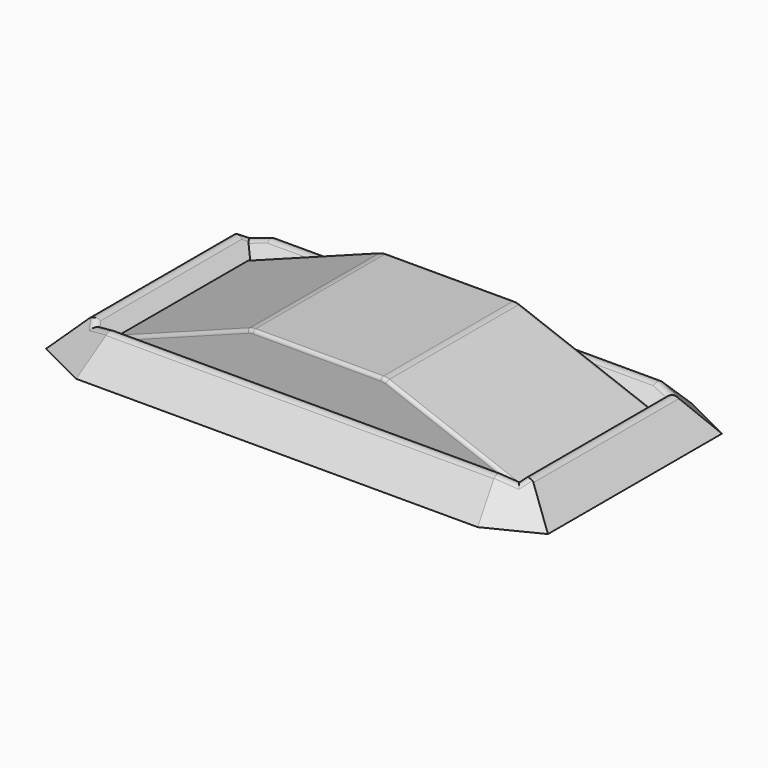
from build123d import *

# Parameters (mm, degrees)
F0_W         = 30.48
F0_H         = 12.7
F1_DEPTH     = 2.54
F2_T1_DEPTH  = 34.8362243683
F3_SIZE      = 2.53999
F4_SIZE      = 2.53999
F5_T4_DEPTH  = 37.0120747894
F5_T10_DEPTH = 19.2320747894
F5_T16_DEPTH = 37.0120747894
F5_T22_DEPTH = 19.2320747894
F6_DEPTH     = 5.08
F7_SIZE2     = 3.80999
F7_SIZE      = 10.15999
F8_T1_DEPTH  = 12.31902
F8_T6_DEPTH  = 12.565371882
F8_T12_DEPTH = 12.565371882
F8_T18_DEPTH = 12.565371882
F8_T24_DEPTH = 12.565371882
F9_T1_DEPTH  = 12.7000000001
F9_T4_ANGLE  = 20.556014319
F9_T6_ANGLE  = 20.556014319
F9_T8_ANGLE  = 20.556014319
F9_T10_ANGLE = 20.556014319
F10_R        = 0.508


# Not quite as in the source:
# - a fillet or chamfer that OpenCascade refuses, or shapes differently, is made with other operations: its cross-section is extruded or revolved along the edge and cut away or added
# - a fillet or chamfer is up to 0.001 mm smaller than in the source, because OpenCascade refuses the exact size


with BuildPart() as f1:
    # F0 (on Top) → F1 (new body)
    with BuildSketch(Plane.XY):
        Polygon((-11.5051504266, -16.4258122915), (-41.9851504266, -16.4258122915), (-47.0651499927, -18.9658166862), (-47.0651499927, -34.2058166862), (-41.9851488709, -36.7458122915), (-11.5051488709, -36.7458122915), (-6.4251502044, -34.2058166862), (-6.4251502044, -18.9658166862), align=None)
        with Locations((-26.7451504266, -26.5858122915)):
            Rectangle(F0_W, F0_H, mode=Mode.SUBTRACT)
    extrude(amount=F1_DEPTH)

    # F2: chamfer of 3.81 on 2 edges, made by hand

    # F2_s2 → F2_t1 (cut)
    with BuildSketch(Plane.XZ.offset(9.167704502)):
        Polygon((-47.0651499927, -1.27), (-43.2551499927, 2.54), (-47.0651499927, 2.54), align=None)
        Polygon((-6.4251502044, -1.27), (-10.2351502044, 2.54), (-6.4251502044, 2.54), align=None)
    extrude(amount=F2_T1_DEPTH, mode=Mode.SUBTRACT)

    # F3 (size 2.54 in the source; OpenCascade refuses exactly that, so slightly less here)
    f3_edges = [f1.edges().sort_by_distance(p)[0] for p in [
        (-42.620149, -36.428313, 2.54),
        (-42.62015, -16.743313, 2.54),
        (-10.87015, -16.743313, 2.54),
        (-10.87015, -36.428313, 2.54),
    ]]
    chamfer(f3_edges, length=F3_SIZE)

    # F4 (size 2.54 in the source; OpenCascade refuses exactly that, so slightly less here)
    f4_edges = [f1.edges().sort_by_distance(p)[0] for p in [
        (-26.745148, -36.745812, 2.54),
        (-26.745151, -16.425812, 2.54),
    ]]
    chamfer(f4_edges, length=F4_SIZE)

    # F5: chamfer of 1.27 on 4 edges, made by hand


with BuildPart() as f5_tool2:
    # F5_s3 → F5_t4 (new body)
    with BuildSketch(Plane.YZ.offset(-45.2511878213)):
        Polygon((-18.9658122915, 2.54), (-20.2358122915, 1.27), (-20.2358122915, 2.54), align=None)
    extrude(amount=F5_T4_DEPTH)

    split(bisect_by=Plane(origin=(-6.3875752133, 0, 6.3875752133), x_dir=(0, 1, 0), z_dir=(-0.7071067812, 0, 0.7071067812)), keep=Keep.TOP)

    split(bisect_by=Plane(origin=(-20.3575752133, 0, -20.3575752133), x_dir=(0, 1, 0), z_dir=(0.7071067812, 0, 0.7071067812)), keep=Keep.TOP)


with BuildPart() as f1_1:
    add(f1.part)

    # F5_t1: cut F5_tool2
    add(f5_tool2.part, mode=Mode.SUBTRACT)


with BuildPart() as f5_tool8:
    # F5_s9 → F5_t10 (new body)
    with BuildSketch(Plane.XZ.offset(36.2018496862)):
        Polygon((-43.2551504266, 2.54), (-41.9851504266, 1.27), (-41.9851504266, 2.54), align=None)
    extrude(amount=-F5_T10_DEPTH)

    split(bisect_by=Plane(origin=(0, -15.8329061458, -15.8329061458), x_dir=(1, 0, 0), z_dir=(0, 0.7071067812, 0.7071067812)), keep=Keep.TOP)

    split(bisect_by=Plane(origin=(0, -10.7529061458, 10.7529061458), x_dir=(1, 0, 0), z_dir=(0, -0.7071067812, 0.7071067812)), keep=Keep.TOP)


with BuildPart() as f1_2:
    add(f1_1.part)

    # F5_t7: cut F5_tool8
    add(f5_tool8.part, mode=Mode.SUBTRACT)


with BuildPart() as f5_tool14:
    # F5_s15 → F5_t16 (new body)
    with BuildSketch(Plane.YZ.offset(-8.2391130319)):
        Polygon((-34.2058122915, 2.54), (-32.9358122915, 1.27), (-32.9358122915, 2.54), align=None)
    extrude(amount=-F5_T16_DEPTH)

    split(bisect_by=Plane(origin=(-6.3875752133, 0, 6.3875752133), x_dir=(0, 1, 0), z_dir=(-0.7071067812, 0, 0.7071067812)), keep=Keep.TOP)

    split(bisect_by=Plane(origin=(-20.3575752133, 0, -20.3575752133), x_dir=(0, 1, 0), z_dir=(0.7071067812, 0, 0.7071067812)), keep=Keep.TOP)


with BuildPart() as f1_3:
    add(f1_2.part)

    # F5_t13: cut F5_tool14
    add(f5_tool14.part, mode=Mode.SUBTRACT)


with BuildPart() as f5_tool20:
    # F5_s21 → F5_t22 (new body)
    with BuildSketch(Plane.XZ.offset(16.9697748968)):
        Polygon((-10.2351504266, 2.54), (-11.5051504266, 1.27), (-11.5051504266, 2.54), align=None)
    extrude(amount=F5_T22_DEPTH)

    split(bisect_by=Plane(origin=(0, -15.8329061458, -15.8329061458), x_dir=(1, 0, 0), z_dir=(0, 0.7071067812, 0.7071067812)), keep=Keep.TOP)

    split(bisect_by=Plane(origin=(0, -10.7529061458, 10.7529061458), x_dir=(1, 0, 0), z_dir=(0, -0.7071067812, 0.7071067812)), keep=Keep.TOP)


with BuildPart() as f1_4:
    add(f1_3.part)

    # F5_t19: cut F5_tool20
    add(f5_tool20.part, mode=Mode.SUBTRACT)

    # F0 (on Top) → F6 (join)
    with BuildSketch(Plane.XY):
        with Locations((-26.7451504266, -26.5858122915)):
            Rectangle(F0_W, F0_H)
    extrude(amount=F6_DEPTH)

    # F7 (size 10.16 and 3.81 in the source; OpenCascade refuses exactly that, so slightly less here)
    f7_edges = [f1_4.edges().sort_by_distance(p)[0] for p in [
        (-41.98515, -26.585812, 5.08),
        (-11.50515, -26.585812, 5.08),
    ]]
    f7_side = f1_4.faces().sort_by_distance((-26.74515, -26.585812, 5.08))[0]
    chamfer(f7_edges, length=F7_SIZE, length2=F7_SIZE2, reference=f7_side)

    # F8: fillet of radius 0.254 on 6 edges, made by hand

    # F8_s2 → F8_t1 (cut)
    with BuildSketch(Plane.YZ.offset(-32.9046604266)):
        with BuildLine():
            ThreePointArc((-32.9358122915, 4.826), (-32.8614174139, 5.0056051224), (-32.6818122915, 5.08))
            Line((-32.6818122915, 5.08), (-32.9358122915, 5.08))
            Line((-32.9358122915, 5.08), (-32.9358122915, 4.826))
        make_face()
        with BuildLine():
            ThreePointArc((-20.4898122915, 5.08), (-20.3102071691, 5.0056051224), (-20.2358122915, 4.826))
            Line((-20.2358122915, 4.826), (-20.2358122915, 5.08))
            Line((-20.2358122915, 5.08), (-20.4898122915, 5.08))
        make_face()
    extrude(amount=F8_T1_DEPTH, mode=Mode.SUBTRACT)


with BuildPart() as f8_tool4:
    # F8_s5 → F8_t6 (new body)
    with BuildSketch(Plane(origin=(-21.6750058731, 0, 8.1281138689), x_dir=(0, 1, 0), z_dir=(0.9363293669, 0, -0.3511229366))):
        with BuildLine():
            ThreePointArc((-32.9358122915, -3.1045745446), (-32.8614174139, -2.9249694222), (-32.6818122915, -2.8505745446))
            Line((-32.6818122915, -2.8505745446), (-32.9358122915, -2.8505745446))
            Line((-32.9358122915, -2.8505745446), (-32.9358122915, -3.1045745446))
        make_face()
    extrude(amount=F8_T6_DEPTH)

    split(bisect_by=Plane(origin=(0, -15.8329061457, -15.8329061457), x_dir=(1, 0, 0), z_dir=(0, 0.7071067812, 0.7071067812)), keep=Keep.TOP)

    split(bisect_by=Plane(origin=(-6.3875752133, 0, 6.3875752133), x_dir=(0, 1, 0), z_dir=(-0.7071067812, 0, 0.7071067812)), keep=Keep.TOP)


with BuildPart() as f1_5:
    add(f1_4.part)

    # F8_t3: cut F8_tool4
    add(f8_tool4.part, mode=Mode.SUBTRACT)


with BuildPart() as f8_tool10:
    # F8_s11 → F8_t12 (new body)
    with BuildSketch(Plane(origin=(-25.2206193231, 0, -9.4577167315), x_dir=(0, 1, 0), z_dir=(-0.9363293669, 0, -0.3511229366))):
        with BuildLine():
            ThreePointArc((-32.9358122915, -15.6770969711), (-32.8614174139, -15.8567020935), (-32.6818122915, -15.9310969711))
            Line((-32.6818122915, -15.9310969711), (-32.9358122915, -15.9310969711))
            Line((-32.9358122915, -15.9310969711), (-32.9358122915, -15.6770969711))
        make_face()
    extrude(amount=F8_T12_DEPTH)

    split(bisect_by=Plane(origin=(0, -15.8329061457, -15.8329061457), x_dir=(1, 0, 0), z_dir=(0, 0.7071067812, 0.7071067812)), keep=Keep.TOP)

    split(bisect_by=Plane(origin=(-20.3575752133, 0, -20.3575752133), x_dir=(0, 1, 0), z_dir=(0.7071067812, 0, 0.7071067812)), keep=Keep.TOP)


with BuildPart() as f1_6:
    add(f1_5.part)

    # F8_t9: cut F8_tool10
    add(f8_tool10.part, mode=Mode.SUBTRACT)


with BuildPart() as f8_tool16:
    # F8_s17 → F8_t18 (new body)
    with BuildSketch(Plane(origin=(-25.2206193231, 0, -9.4577167315), x_dir=(0, 1, 0), z_dir=(-0.9363293669, 0, -0.3511229366))):
        with BuildLine():
            ThreePointArc((-20.4898122915, -15.9310969711), (-20.3102071691, -15.8567020935), (-20.2358122915, -15.6770969711))
            Line((-20.2358122915, -15.6770969711), (-20.2358122915, -15.9310969711))
            Line((-20.2358122915, -15.9310969711), (-20.4898122915, -15.9310969711))
        make_face()
    extrude(amount=F8_T18_DEPTH)

    split(bisect_by=Plane(origin=(-20.3575752133, 0, -20.3575752133), x_dir=(0, 1, 0), z_dir=(0.7071067812, 0, 0.7071067812)), keep=Keep.TOP)

    split(bisect_by=Plane(origin=(0, -10.7529061458, 10.7529061458), x_dir=(1, 0, 0), z_dir=(0, -0.7071067812, 0.7071067812)), keep=Keep.TOP)


with BuildPart() as f1_7:
    add(f1_6.part)

    # F8_t15: cut F8_tool16
    add(f8_tool16.part, mode=Mode.SUBTRACT)


with BuildPart() as f8_tool22:
    # F8_s23 → F8_t24 (new body)
    with BuildSketch(Plane(origin=(-21.6750058731, 0, 8.1281138689), x_dir=(0, 1, 0), z_dir=(0.9363293669, 0, -0.3511229366))):
        with BuildLine():
            ThreePointArc((-20.4898122915, -2.8505745446), (-20.3102071691, -2.9249694222), (-20.2358122915, -3.1045745446))
            Line((-20.2358122915, -3.1045745446), (-20.2358122915, -2.8505745446))
            Line((-20.2358122915, -2.8505745446), (-20.4898122915, -2.8505745446))
        make_face()
    extrude(amount=F8_T24_DEPTH)

    split(bisect_by=Plane(origin=(-6.3875752133, 0, 6.3875752133), x_dir=(0, 1, 0), z_dir=(-0.7071067812, 0, 0.7071067812)), keep=Keep.TOP)

    split(bisect_by=Plane(origin=(0, -10.7529061458, 10.7529061458), x_dir=(1, 0, 0), z_dir=(0, -0.7071067812, 0.7071067812)), keep=Keep.TOP)


with BuildPart() as f1_8:
    add(f1_7.part)

    # F8_t21: cut F8_tool22
    add(f8_tool22.part, mode=Mode.SUBTRACT)

    # F9: fillet of radius 1.27 on 2 edges, made by hand

    # F9_s2 → F9_t1 (cut)
    with BuildSketch(Plane.XZ.offset(20.2358122914)):
        with BuildLine():
            ThreePointArc((-31.5948658615, 5.08), (-31.8214650275, 5.0596210698), (-32.040791991, 4.999138296))
            Line((-32.040791991, 4.999138296), (-31.8251604266, 5.08))
            Line((-31.8251604266, 5.08), (-31.5948658615, 5.08))
        make_face()
        with BuildLine():
            ThreePointArc((-21.4495088623, 4.999138296), (-21.6688358257, 5.0596210698), (-21.8954349918, 5.08))
            Line((-21.8954349918, 5.08), (-21.6651404266, 5.08))
            Line((-21.6651404266, 5.08), (-21.4495088623, 4.999138296))
        make_face()
    extrude(amount=F9_T1_DEPTH, mode=Mode.SUBTRACT)

    # F9_s3 → F9_t4 (revolve, cut)
    with BuildSketch(Plane(origin=(-20.4486067571, 0, 7.6682149548), x_dir=(0, 1, 0), z_dir=(0.9363293669, 0, -0.3511229366))):
        with BuildLine():
            ThreePointArc((-32.9358122915, -3.1045745447), (-32.8614174139, -2.9249694222), (-32.6818122914, -2.8505745446))
            Line((-32.6818122914, -2.8505745446), (-32.9358122915, -2.8505745446))
            Line((-32.9358122915, -2.8505745446), (-32.9358122915, -3.1045745447))
        make_face()
    revolve(axis=Axis((-21.8954349918, -32.9358122915, 3.81), (0, -1, 0)), revolution_arc=F9_T4_ANGLE, mode=Mode.SUBTRACT)

    # F9_s5 → F9_t6 (revolve, cut)
    with BuildSketch(Plane.YZ.offset(-21.8954349918)):
        with BuildLine():
            ThreePointArc((-20.2358122915, 4.8259999999), (-20.3102071691, 5.0056051224), (-20.4898122916, 5.08))
            Line((-20.4898122916, 5.08), (-20.2358122915, 5.08))
            Line((-20.2358122915, 5.08), (-20.2358122915, 4.8259999999))
        make_face()
    revolve(axis=Axis((-21.8954349918, -20.2358122915, 3.81), (0, 1, 0)), revolution_arc=F9_T6_ANGLE, mode=Mode.SUBTRACT)

    # F9_s7 → F9_t8 (revolve, cut)
    with BuildSketch(Plane(origin=(-26.4470184391, 0, -9.9176156456), x_dir=(0, 1, 0), z_dir=(-0.9363293669, 0, -0.3511229366))):
        with BuildLine():
            ThreePointArc((-20.2358122915, -15.6770969711), (-20.3102071691, -15.8567020935), (-20.4898122916, -15.9310969711))
            Line((-20.4898122916, -15.9310969711), (-20.2358122915, -15.9310969711))
            Line((-20.2358122915, -15.9310969711), (-20.2358122915, -15.6770969711))
        make_face()
    revolve(axis=Axis((-31.5948658615, -20.2358122915, 3.81), (0, 1, 0)), revolution_arc=F9_T8_ANGLE, mode=Mode.SUBTRACT)

    # F9_s9 → F9_t10 (revolve, cut)
    with BuildSketch(Plane.YZ.offset(-31.5948658615)):
        with BuildLine():
            ThreePointArc((-32.9358122915, 4.8259999999), (-32.8614174139, 5.0056051224), (-32.6818122914, 5.08))
            Line((-32.6818122914, 5.08), (-32.9358122915, 5.08))
            Line((-32.9358122915, 5.08), (-32.9358122915, 4.8259999999))
        make_face()
    revolve(axis=Axis((-31.5948658615, -32.9358122915, 3.81), (0, -1, 0)), revolution_arc=F9_T10_ANGLE, mode=Mode.SUBTRACT)

    # F10
    f10_edges = [f1_8.edges().sort_by_distance(p)[0] for p in [
        (-43.25515, -26.585814, 2.54),
        (-43.07662, -19.611741, 2.36147),
        (-42.141814, -19.144338, 2.36147),
        (-26.74515, -18.965802, 2.54),
        (-11.348486, -19.144338, 2.36147),
        (-10.413681, -19.611741, 2.36147),
        (-10.23515, -26.585815, 2.54),
        (-11.348484, -34.027288, 2.36147),
        (-10.41368, -33.559886, 2.36147),
        (-26.745149, -34.205822, 2.54),
        (-43.076621, -33.559886, 2.36147),
        (-41.685355, -34.13504, 2.469228),
        (-42.441621, -33.956511, 2.290698),
    ]]
    fillet(f10_edges, radius=F10_R)


solid = f1_8.part
